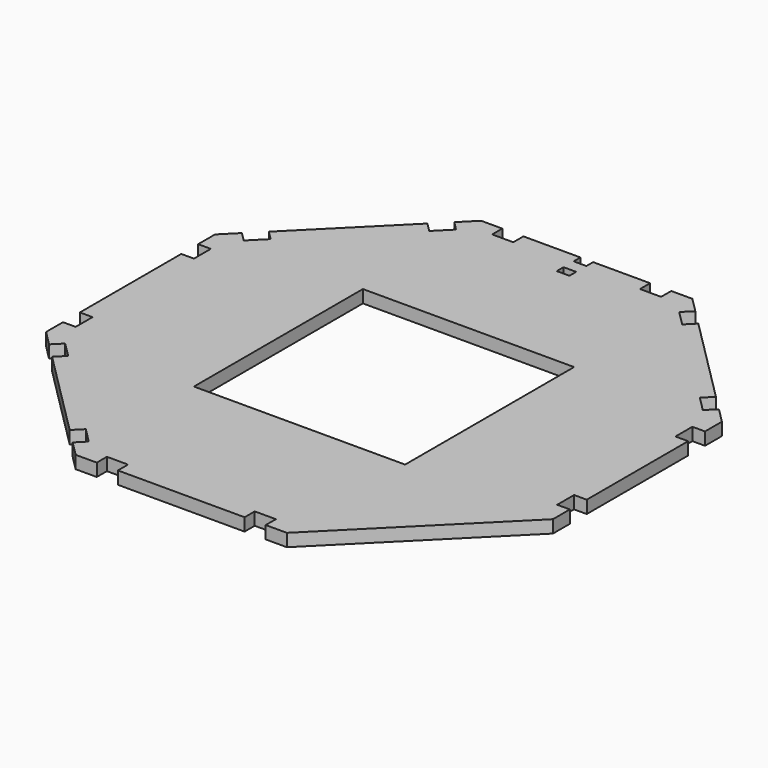
from build123d import *

# Parameters (mm, degrees)
F0_W     = 1270
F0_H     = 1270
F0_W_2   = 38.1
F0_H_2   = 76.2
F1_DEPTH = 25.4
F2_DEPTH = 76.2


# Not quite as in the source:
# - ends of sketch curves that miss each other by under 0.0002 mm in the source are joined


with BuildPart() as f1:
    # F0 (on Top) → F1 (new body)
    with BuildSketch(Plane.XY):
        Polygon((-1434.1974387893, 724.8025612107), (-1524, 635), (-1524, 508), (-1447.8, 508), (-1447.8, 381), (-1524, 381), (-1524, -381), (-1447.8, -381), (-1447.8, -508), (-1524, -508), (-1524, -635), (-1434.1974387893, -724.8025612107), (-1380.3159020629, -670.9210244843), (-1290.5133408522, -760.723585695), (-1344.3948775786, -814.6051224214), (-814.6051224214, -1344.3948775786), (-760.723585695, -1290.5133408522), (-670.9210244843, -1380.3159020629), (-724.8025612107, -1434.1974387893), (-635, -1524), (-508, -1524), (-508, -1447.8), (-381, -1447.8), (-381, -1524), (0, -1524), (381, -1524), (381, -1447.8), (508, -1447.8), (508, -1524), (635, -1524), (724.8025612107, -1434.1974387893), (670.9210244843, -1380.3159020629), (760.723585695, -1290.5133408522), (814.6051224214, -1344.3948775786), (1344.3948775786, -814.6051224214), (1290.5133408522, -760.723585695), (1380.3159020629, -670.9210244843), (1434.1974387893, -724.8025612107), (1524, -635), (1524, -508), (1447.8, -508), (1447.8, -381), (1524, -381), (1524, 381), (1447.8, 381), (1447.8, 508), (1524, 508), (1524, 635), (1434.1974387893, 724.8025612107), (1380.3159020629, 670.9210244843), (1290.5133408522, 760.723585695), (1344.3948775786, 814.6051224214), (814.6051224214, 1344.3948775786), (760.723585695, 1290.5133408522), (670.9210244843, 1380.3159020629), (724.8025612107, 1434.1974387893), (635, 1524), (508, 1524), (508, 1447.8), (381, 1447.8), (381, 1524), (38.1, 1524), (38.1, 1473.2), (38.1, 1397), (38.1, 1346.2), (-38.1, 1346.2), (-38.1, 1397), (-38.1, 1473.2), (-38.1, 1523.9999635696), (-381, 1524), (-381, 1447.8), (-508, 1447.8), (-508, 1524), (-635, 1524), (-724.8025612107, 1434.1974387893), (-670.9210244843, 1380.3159020629), (-760.723585695, 1290.5133408522), (-814.6051224214, 1344.3948775786), (-1344.3948775786, 814.6051224214), (-1290.5133408522, 760.723585695), (-1380.3159020629, 670.9210244843), align=None)
        Rectangle(F0_W, F0_H, mode=Mode.SUBTRACT)
        with Locations((-19.05, 1435.1)):
            Rectangle(F0_W_2, F0_H_2)
        with Locations((19.05, 1435.1)):
            Rectangle(F0_W_2, F0_H_2)
        Polygon((670.9210244843, -1380.3159020629), (724.8025612107, -1434.1974387893), (814.6051224214, -1344.3948775786), (760.723585695, -1290.5133408522), align=None)
        Polygon((1290.5133408522, -760.723585695), (1344.3948775786, -814.6051224214), (1434.1974387893, -724.8025612107), (1380.3159020629, -670.9210244843), align=None)
    extrude(amount=F1_DEPTH)

    # F0 (on Top) → F2 (join)
    with BuildSketch(Plane.XY):
        Polygon((-1434.1974387893, 724.8025612107), (-1524, 635), (-1524, 508), (-1447.8, 508), (-1447.8, 381), (-1524, 381), (-1524, -381), (-1447.8, -381), (-1447.8, -508), (-1524, -508), (-1524, -635), (-1434.1974387893, -724.8025612107), (-1380.3159020629, -670.9210244843), (-1290.5133408522, -760.723585695), (-1344.3948775786, -814.6051224214), (-814.6051224214, -1344.3948775786), (-760.723585695, -1290.5133408522), (-670.9210244843, -1380.3159020629), (-724.8025612107, -1434.1974387893), (-635, -1524), (-508, -1524), (-508, -1447.8), (-381, -1447.8), (-381, -1524), (0, -1524), (381, -1524), (381, -1447.8), (508, -1447.8), (508, -1524), (635, -1524), (724.8025612107, -1434.1974387893), (670.9210244843, -1380.3159020629), (760.723585695, -1290.5133408522), (814.6051224214, -1344.3948775786), (1344.3948775786, -814.6051224214), (1290.5133408522, -760.723585695), (1380.3159020629, -670.9210244843), (1434.1974387893, -724.8025612107), (1524, -635), (1524, -508), (1447.8, -508), (1447.8, -381), (1524, -381), (1524, 381), (1447.8, 381), (1447.8, 508), (1524, 508), (1524, 635), (1434.1974387893, 724.8025612107), (1380.3159020629, 670.9210244843), (1290.5133408522, 760.723585695), (1344.3948775786, 814.6051224214), (814.6051224214, 1344.3948775786), (760.723585695, 1290.5133408522), (670.9210244843, 1380.3159020629), (724.8025612107, 1434.1974387893), (635, 1524), (508, 1524), (508, 1447.8), (381, 1447.8), (381, 1524), (38.1, 1524), (38.1, 1473.2), (38.1, 1397), (38.1, 1346.2), (-38.1, 1346.2), (-38.1, 1397), (-38.1, 1473.2), (-38.1, 1523.9999635696), (-381, 1524), (-381, 1447.8), (-508, 1447.8), (-508, 1524), (-635, 1524), (-724.8025612107, 1434.1974387893), (-670.9210244843, 1380.3159020629), (-760.723585695, 1290.5133408522), (-814.6051224214, 1344.3948775786), (-1344.3948775786, 814.6051224214), (-1290.5133408522, 760.723585695), (-1380.3159020629, 670.9210244843), align=None)
        Rectangle(F0_W, F0_H, mode=Mode.SUBTRACT)
        with Locations((-19.05, 1435.1)):
            Rectangle(F0_W_2, F0_H_2)
        with Locations((19.05, 1435.1)):
            Rectangle(F0_W_2, F0_H_2)
        Polygon((670.9210244843, -1380.3159020629), (724.8025612107, -1434.1974387893), (814.6051224214, -1344.3948775786), (760.723585695, -1290.5133408522), align=None)
        Polygon((1290.5133408522, -760.723585695), (1344.3948775786, -814.6051224214), (1434.1974387893, -724.8025612107), (1380.3159020629, -670.9210244843), align=None)
    extrude(amount=F2_DEPTH)


solid = f1.part
